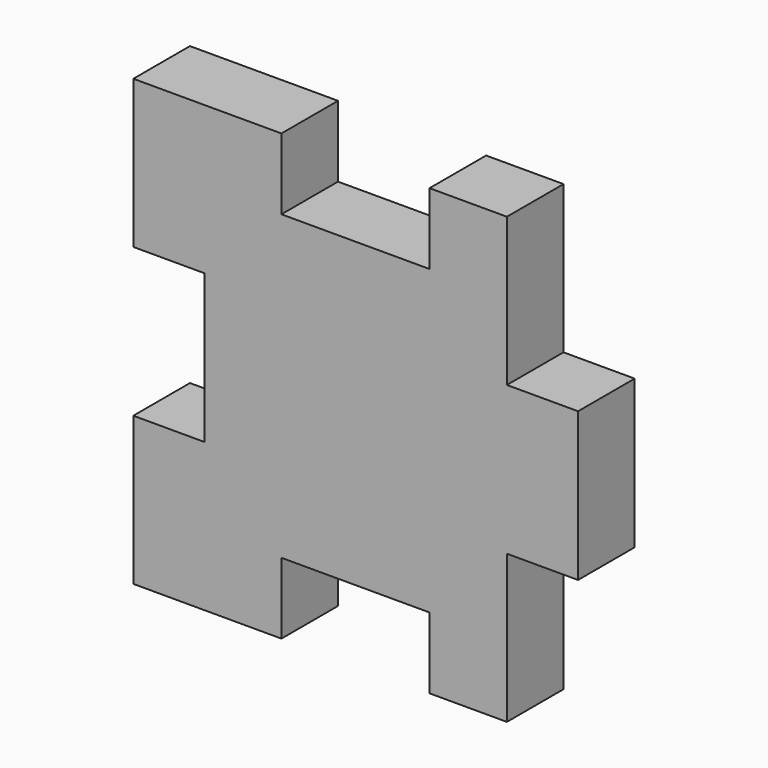
from build123d import *

# Parameters (mm, degrees)
F1_DEPTH     = 2.032
F3_TEXT_SIZE = 7.6814534605
F4_DEPTH     = 0.508


# Not quite as in the source:
# - Text() gives the source's letters only with a copy of the font that has no kerning and outlines rounded to 1/6400 em; it was checked with that copy


with BuildPart() as f1:
    # F0 (on Front) → F1 (new body)
    with BuildSketch(Plane.XZ):
        Polygon((-10.9897290399, 29.0234165891), (-10.9897290399, 26.8898165891), (-10.9897290399, 24.7562165891), (-13.0344290399, 24.7562165891), (-13.0344290399, 20.5017165891), (-8.7799290399, 20.5017165891), (-8.7799290399, 22.5464165891), (-4.5254290399, 22.5464165891), (-4.5254290399, 20.5017165891), (-2.3029290399, 20.5017165891), (-2.3029290399, 24.7562165891), (-0.2582290399, 24.7562165891), (-0.2582290399, 29.0234165891), (-2.3029290399, 29.0234165891), (-2.3029290399, 33.2779165891), (-4.5254290399, 33.2779165891), (-4.5254290399, 31.2332165891), (-8.7799290399, 31.2332165891), (-8.7799290399, 33.2779165891), (-13.0344290399, 33.2779165891), (-13.0344290399, 29.0234165891), align=None)
    extrude(amount=F1_DEPTH)

    # F3 (on offset) → F4 (cut)
    with BuildSketch(Plane.XZ.offset(4.064)):
        with Locations((-9.1051172327, 24.3420478711)):
            Text('N', F3_TEXT_SIZE, font='Open Sans', text_align=(TextAlign.LEFT, TextAlign.BOTTOM))
    extrude(amount=-F4_DEPTH, mode=Mode.SUBTRACT)


solid = f1.part
